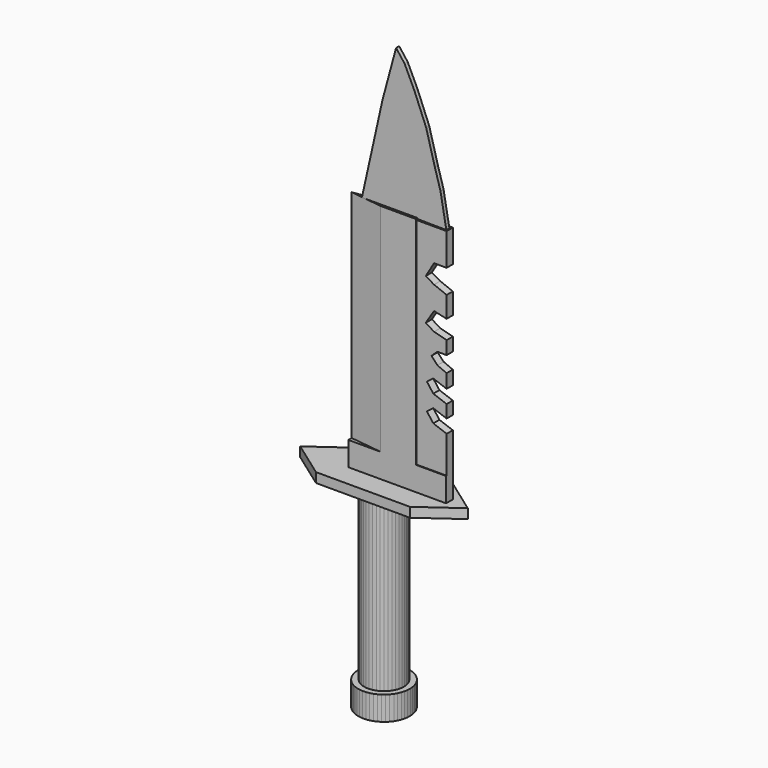
from build123d import *

# Parameters (mm, degrees)
F1_DEPTH  = 12.7
F3_DEPTH  = 88.9
F4_W      = 49.5914556086
F4_H      = 27.8375800699
F5_DEPTH  = 5.08
F7_DEPTH  = 5.08
F8_DEPTH  = 5.08
F9_W      = 51.6053037718
F9_H      = 4.4333104743
F10_DEPTH = 12.7
F11_W     = 18.5319427401
F11_H     = 4.4333104743
F12_DEPTH = 114.3
F14_DEPTH = 114.3
F16_DEPTH = 4.064
F18_DEPTH = 1.016
F19_DEPTH = 1.016


# Not quite as in the source:
# - a length typed as a fraction of an inch, garbled in the dataset ("3 / 203.2 mm" for 3/8 in), is restored


with BuildPart() as f1:
    # F0 (on Top) → F1 (new body)
    with BuildSketch(Plane.XY):
        Polygon((7.6455804064, -11.218967169), (8.9914021538, -10.1722569471), (10.195424118, -8.9651241566), (11.2386581535, -7.6166060026), (12.1046518362, -6.147969422), (12.7797479285, -4.582375691), (13.2532997617, -2.9445151579), (13.5178391405, -1.2602178619), (13.569194121, 0.4439538226), (13.4065548043, 2.1411240902), (13.0324861096, 3.8045275518), (12.4528873238, 5.4079313412), (11.6768990658, 6.9260488228), (10.7167591342, 8.334938377), (9.5876095091, 9.612380974), (8.3072575547, 10.7382305809), (6.8958951862, 11.6947318768), (5.3757804312, 12.4668002649), (3.7708864074, 13.0422597655), (2.1065232524, 13.4120350386), (0.4089389673, 13.5702945071), (-1.2950945296, 13.5145423248), (-2.9787036121, 13.2456577368), (-4.6153367593, 12.7678812137), (-6.1791832887, 12.0887475767), (-7.6455804064, 11.218967169), (-8.9914021538, 10.1722569471), (-10.195424118, 8.9651241566), (-11.2386581535, 7.6166060026), (-12.1046518362, 6.147969422), (-12.7797479285, 4.582375691), (-13.2532997617, 2.9445151579), (-13.5178391405, 1.2602178619), (-13.569194121, -0.4439538226), (-13.4065548043, -2.1411240902), (-13.0324861096, -3.8045275518), (-12.4528873238, -5.4079313412), (-11.6768990658, -6.9260488228), (-10.7167591342, -8.334938377), (-9.5876095091, -9.612380974), (-8.3072575547, -10.7382305809), (-6.8958951862, -11.6947318768), (-5.3757804312, -12.4668002649), (-3.7708864074, -13.0422597655), (-2.1065232524, -13.4120350386), (-0.4089389673, -13.5702945071), (1.2950945296, -13.5145423248), (2.9787036121, -13.2456577368), (4.6153367593, -12.7678812137), (6.1791832887, -12.0887475767), align=None)
    extrude(amount=F1_DEPTH)

    # F2 (on face) → F3 (join)
    with BuildSketch(Plane.XY.offset(12.7)):
        Polygon((2.1904929984, -10.2495944917), (3.7669142259, -9.7807363749), (5.2505815234, -9.0710440681), (6.6049620782, -8.1379925514), (7.796706546, -7.0045566495), (8.7964702228, -5.6986453162), (9.5796356089, -4.2524144224), (10.1269185734, -2.7014749726), (10.4248431933, -1.0840162433), (10.4660735757, 0.5601345635), (10.2495944917, 2.1904929984), (9.7807363749, 3.7669142259), (9.0710440681, 5.2505815234), (8.1379925514, 6.6049620782), (7.0045566495, 7.796706546), (5.6986453162, 8.7964702228), (4.2524144224, 9.5796356089), (2.7014749726, 10.1269185734), (1.0840162433, 10.4248431933), (-0.5601345635, 10.4660735757), (-2.1904929984, 10.2495944917), (-3.7669142259, 9.7807363749), (-5.2505815234, 9.0710440681), (-6.6049620782, 8.1379925514), (-7.796706546, 7.0045566495), (-8.7964702228, 5.6986453162), (-9.5796356089, 4.2524144224), (-10.1269185734, 2.7014749726), (-10.4248431933, 1.0840162433), (-10.4660735757, -0.5601345635), (-10.2495944917, -2.1904929984), (-9.7807363749, -3.7669142259), (-9.0710440681, -5.2505815234), (-8.1379925514, -6.6049620782), (-7.0045566495, -7.796706546), (-5.6986453162, -8.7964702228), (-4.2524144224, -9.5796356089), (-2.7014749726, -10.1269185734), (-1.0840162433, -10.4248431933), (0.5601345635, -10.4660735757), align=None)
    extrude(amount=F3_DEPTH)

    # F4 (on face) → F5 (join)
    with BuildSketch(Plane.XY.offset(101.6)):
        Rectangle(F4_W, F4_H)
    extrude(amount=F5_DEPTH)

    # F6 (on face) → F7 (join)
    with BuildSketch(Plane(origin=(0, 0, 101.6), x_dir=(1, 0, 0), z_dir=(0, 0, -1))):
        Polygon((-44.2462861538, 0), (-24.7957278043, -13.9187900349), (-24.7957278043, 13.9187900349), align=None)
    extrude(amount=-F7_DEPTH)

    # F6 (on face) → F8 (join)
    with BuildSketch(Plane(origin=(0, 0, 101.6), x_dir=(1, 0, 0), z_dir=(0, 0, -1))):
        Polygon((24.7957278043, 13.9187900349), (24.7957278043, -13.9187900349), (44.2214161158, 0), align=None)
    extrude(amount=-F8_DEPTH)

    # F9 (on face) → F10 (join)
    with BuildSketch(Plane.XY.offset(106.68)):
        with Locations((8.7059200741, 0.0440463773)):
            Rectangle(F9_W, F9_H)
    extrude(amount=F10_DEPTH)

    # F11 (on face) → F12 (join)
    with BuildSketch(Plane.XY.offset(119.38)):
        with Locations((9.26597137, 0.0440463773)):
            Rectangle(F11_W, F11_H)
    extrude(amount=F12_DEPTH)

    # F13 (on face) → F14 (join)
    with BuildSketch(Plane.XY.offset(119.38)):
        Polygon((0, -2.1726088598), (0, 2.2607016144), (-17.0967318118, 0), align=None)
    extrude(amount=F14_DEPTH)

    # F15 (on face) → F16 (join)
    with BuildSketch(Plane(origin=(0, 2.2607016144, 0), x_dir=(-1, 0, 0), z_dir=(0, 1, 0))):
        Polygon((-34.50857196, 124.4318857789), (-34.50857196, 119.38), (-18.5319427401, 119.38), (-18.5319427401, 233.0740690231), (-34.50857196, 233.0740690231), (-34.50857196, 216.0275018554), (-27.85702236, 216.0275018554), (-23.4947055578, 208.6254060268), (-27.85702236, 206.0545384884), (-34.50857196, 203.4297866207), (-34.50857196, 192.3147596109), (-27.85702236, 193.8075326945), (-23.4947055578, 186.8935078382), (-27.85702236, 184.1411590576), (-34.50857196, 182.4075117771), (-34.50857196, 175.4231682831), (-29.6370955184, 175.4231682831), (-26.5028076246, 172.5162565708), (-29.6370955184, 169.1368073225), (-34.50857196, 167.0584704934), (-34.50857196, 159.7376912832), (-27.4633802474, 162.3028325299), (-24.0699224556, 159.7376912832), (-27.4633802474, 155.2484430598), (-34.50857196, 152.6833018131), (-34.50857196, 145.9243744612), (-27.4633802474, 148.4895157079), (-24.0699224556, 145.9243744612), (-27.4633802474, 141.4351262377), (-34.50857196, 138.869984991), (-34.50857196, 131.7707747221), align=None)
    extrude(amount=-F16_DEPTH)

    # F17 (on Front) → F18 (join)
    with BuildSketch(Plane.XZ):
        Polygon((-10.8600538224, 233.6585074663), (33.719830215, 233.0019772053), (30.6109376252, 250.2144873142), (27.6256743819, 260.3836655617), (23.0536255985, 277.1858274937), (16.9042795897, 292.2313511372), (11.6809960455, 303.2293915749), (7.1772807278, 309.0918958187), (0, 282.517939806), align=None)
    extrude(amount=F18_DEPTH)

    # F17 (on Front) → F19 (join)
    with BuildSketch(Plane.XZ):
        Polygon((-10.8600538224, 233.6585074663), (33.719830215, 233.0019772053), (30.6109376252, 250.2144873142), (27.6256743819, 260.3836655617), (23.0536255985, 277.1858274937), (16.9042795897, 292.2313511372), (11.6809960455, 303.2293915749), (7.1772807278, 309.0918958187), (0, 282.517939806), align=None)
    extrude(amount=-F19_DEPTH)


solid = f1.part
